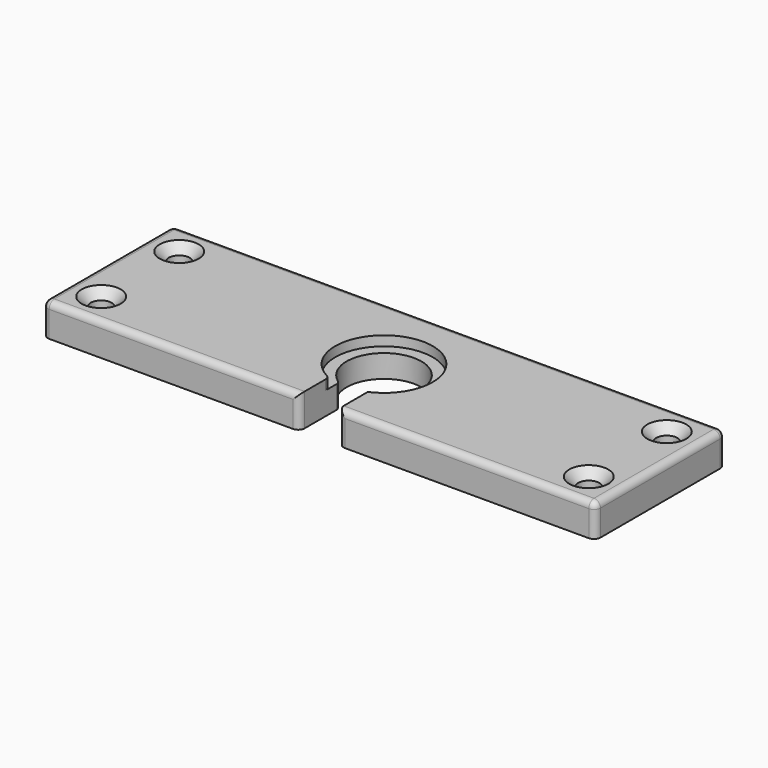
from build123d import *

# Parameters (mm, degrees)
F0_W            = 170
F0_H            = 50
F0_R            = 11.5
F1_DEPTH        = 10
F2_R            = 3.25
F3_DEPTH        = 10.001
F4_R            = 15
F4_R_2          = 11.5
F5_DEPTH        = 3
F7_DEPTH        = 25
F8_T1_DEPTH     = 20.004828627
F8_T3_DEPTH     = 12.3229236974
F8_T5_DEPTH     = 6.1336823274
F9_T1_DEPTH     = 46
F9_T3_DEPTH     = 166
F9_T5_DEPTH     = 13
F9_T7_DEPTH     = 80.0390459698
F9_T9_DEPTH     = 80.0390459698
F9_S13_W        = 2
F9_S13_H        = 2
F9_T14_DEPTH    = 2
F9_S19_W        = 2
F9_S19_H        = 2
F9_T20_DEPTH    = 2
F9_S25_W        = 2
F9_S25_H        = 2
F9_T26_DEPTH    = 2
F9_S31_W        = 2
F9_S31_H        = 2
F9_T32_DEPTH    = 2
F11_D           = 6.5
F11_DEPTH       = 15
F11_CSINK_D     = 12
F11_CSINK_ANGLE = 90
F11_TIP         = 1.9527970118


# Not quite as in the source:
# - a fillet or chamfer that OpenCascade refuses, or shapes differently, is made with other operations: its cross-section is extruded or revolved along the edge and cut away or added


with BuildPart() as f1:
    # F0 (on Top) → F1 (new body)
    with BuildSketch(Plane.XY):
        Rectangle(F0_W, F0_H)
        Circle(F0_R, mode=Mode.SUBTRACT)
    extrude(amount=F1_DEPTH)

    # F2 (on face) → F3 (cut, through all)
    with BuildSketch(Plane.XY.offset(10)):
        with Locations((-75, 15)):
            Circle(F2_R)
        with Locations((-75, -15)):
            Circle(F2_R)
        with Locations((75, -15)):
            Circle(F2_R)
        with Locations((75, 15)):
            Circle(F2_R)
    extrude(amount=-F3_DEPTH, mode=Mode.SUBTRACT)

    # F4 (on face) → F5 (cut)
    with BuildSketch(Plane.XY.offset(10)):
        Circle(F4_R)
        Circle(F4_R_2, mode=Mode.SUBTRACT)
    extrude(amount=-F5_DEPTH, mode=Mode.SUBTRACT)

    # F6 (on face) → F7 (cut)
    with BuildSketch(Plane.XY.offset(10)):
        with BuildLine():
            Line((-6, -13.7477270849), (-6, -25))
            Line((-6, -25), (6, -25))
            Line((6, -25), (6, -13.7477270849))
            ThreePointArc((6, -13.7477270849), (0, -15), (-6, -13.7477270849))
        make_face()
        with BuildLine():
            Line((-6, -9), (-6, -13.7477270849))
            ThreePointArc((-6, -13.7477270849), (0, -15), (6, -13.7477270849))
            Line((6, -13.7477270849), (6, -9))
            Line((6, -9), (-6, -9))
        make_face()
    extrude(amount=-F7_DEPTH, mode=Mode.SUBTRACT)

    # F8: fillet of radius 2 on 5 edges, made by hand

    # F8_s2 → F8_t1 (cut)
    with BuildSketch(Plane.XY.offset(-5.0024143135)):
        with BuildLine():
            ThreePointArc((-5.9996, -22.9990343146), (-6.5857864376, -24.4142135624), (-8.0009656854, -25.0004))
            Line((-8.0009656854, -25.0004), (-8.0009656854, -25.2005365685))
            ThreePointArc((-8.0009656854, -25.2005365685), (-7.0004828427, -25.2001365685), (-6, -25.2001365685))
            Line((-6, -25.2001365685), (-5.7998634315, -25))
            ThreePointArc((-5.7998634315, -25), (-5.7998634315, -23.9995171573), (-5.7994634315, -22.9990343146))
            Line((-5.7994634315, -22.9990343146), (-5.9996, -22.9990343146))
        make_face()
        with BuildLine():
            ThreePointArc((5.9996, -22.9990343146), (6.5857864376, -24.4142135624), (8.0009656854, -25.0004))
            Line((8.0009656854, -25.0004), (8.0009656854, -25.2005365685))
            ThreePointArc((8.0009656854, -25.2005365685), (7.0004828427, -25.2001365685), (6, -25.2001365685))
            Line((6, -25.2001365685), (5.7998634315, -25))
            ThreePointArc((5.7998634315, -25), (5.7998634315, -23.9995171573), (5.7994634315, -22.9990343146))
            Line((5.7994634315, -22.9990343146), (5.9996, -22.9990343146))
        make_face()
    extrude(amount=F8_T1_DEPTH, mode=Mode.SUBTRACT)

    # F8_s4 → F8_t3 (cut)
    with BuildSketch(Plane.XY.offset(-2.6614618487)):
        with BuildLine():
            ThreePointArc((-6.8152717523, -9.2624441214), (-6.215115784, -9.9716058978), (-5.9996, -10.8752930995))
            Line((-5.9996, -10.8752930995), (-5.79936, -10.8752930995))
            ThreePointArc((-5.79936, -10.8752930995), (-5.79976, -10.3430007673), (-5.79976, -9.8107084352))
            Line((-5.79976, -9.8107084352), (-5.8955269565, -9.6398826737))
            ThreePointArc((-5.8955269565, -9.6398826737), (-6.3019268651, -9.3792480426), (-6.6965989276, -9.1011592236))
            Line((-6.6965989276, -9.1011592236), (-6.8152717523, -9.2624441214))
        make_face()
        with BuildLine():
            ThreePointArc((5.9996, -10.8752930995), (6.215115784, -9.9716058978), (6.8152717523, -9.2624441214))
            Line((6.8152717523, -9.2624441214), (6.6965989276, -9.1011592236))
            ThreePointArc((6.6965989276, -9.1011592236), (6.3019268651, -9.3792480426), (5.8955269565, -9.6398826737))
            Line((5.8955269565, -9.6398826737), (5.79976, -9.8107084352))
            ThreePointArc((5.79976, -9.8107084352), (5.79976, -10.3430007673), (5.79936, -10.8752930995))
            Line((5.79936, -10.8752930995), (5.9996, -10.8752930995))
        make_face()
    extrude(amount=F8_T3_DEPTH, mode=Mode.SUBTRACT)

    # F8_s6 → F8_t5 (cut)
    with BuildSketch(Plane.XY.offset(7)):
        with BuildLine():
            ThreePointArc((-7.0595694154, -13.2344429361), (-6.2849198093, -13.9710342475), (-5.9996, -15.001199952))
            Line((-5.9996, -15.001199952), (-5.79936, -15.001199952))
            ThreePointArc((-5.79936, -15.001199952), (-5.79976, -14.3744635184), (-5.79976, -13.7477270849))
            Line((-5.79976, -13.7477270849), (-5.919904, -13.5642040934))
            ThreePointArc((-5.919904, -13.5642040934), (-6.4476696186, -13.3214283223), (-6.9653263569, -13.0577672345))
            Line((-6.9653263569, -13.0577672345), (-7.0595694154, -13.2344429361))
        make_face()
    extrude(amount=F8_T5_DEPTH, mode=Mode.SUBTRACT)

    # F9: fillet of radius 2 on 9 edges, made by hand

    # F9_s2 → F9_t1 (cut)
    with BuildSketch(Plane.XZ.offset(-23)):
        with BuildLine():
            ThreePointArc((-83, 10), (-84.4142135624, 9.4142135624), (-85, 8))
            Line((-85, 8), (-85, 10))
            Line((-85, 10), (-83, 10))
        make_face()
        with BuildLine():
            ThreePointArc((85, 8), (84.4142135624, 9.4142135624), (83, 10))
            Line((83, 10), (85, 10))
            Line((85, 10), (85, 8))
        make_face()
    extrude(amount=F9_T1_DEPTH, mode=Mode.SUBTRACT)

    # F9_s4 → F9_t3 (cut)
    with BuildSketch(Plane.YZ.offset(-83)):
        with BuildLine():
            ThreePointArc((23, 10), (24.4142135624, 9.4142135624), (25, 8))
            Line((25, 8), (25, 10))
            Line((25, 10), (23, 10))
        make_face()
    extrude(amount=F9_T3_DEPTH, mode=Mode.SUBTRACT)

    # F9_s6 → F9_t5 (cut)
    with BuildSketch(Plane.XY.offset(-5)):
        with BuildLine():
            ThreePointArc((85, -23), (84.4142135624, -24.4142135624), (83, -25))
            Line((83, -25), (85, -25))
            Line((85, -25), (85, -23))
        make_face()
        with BuildLine():
            ThreePointArc((85, 23), (84.4142135624, 24.4142135624), (83, 25))
            Line((83, 25), (85, 25))
            Line((85, 25), (85, 23))
        make_face()
        with BuildLine():
            ThreePointArc((-85, -23), (-84.4142135624, -24.4142135624), (-83, -25))
            Line((-83, -25), (-85, -25))
            Line((-85, -25), (-85, -23))
        make_face()
        with BuildLine():
            ThreePointArc((-85, 23), (-84.4142135624, 24.4142135624), (-83, 25))
            Line((-83, 25), (-85, 25))
            Line((-85, 25), (-85, 23))
        make_face()
    extrude(amount=F9_T5_DEPTH, mode=Mode.SUBTRACT)

    # F9_s8 → F9_t7 (cut)
    with BuildSketch(Plane.YZ.offset(2.9609540302)):
        with BuildLine():
            ThreePointArc((-23, 10), (-24.4142135624, 9.4142135624), (-25, 8))
            Line((-25, 8), (-25, 10))
            Line((-25, 10), (-23, 10))
        make_face()
    extrude(amount=F9_T7_DEPTH, mode=Mode.SUBTRACT)

    # F9_s10 → F9_t9 (cut)
    with BuildSketch(Plane.YZ.offset(-83)):
        with BuildLine():
            ThreePointArc((-23, 10), (-24.4142135624, 9.4142135624), (-25, 8))
            Line((-25, 8), (-25, 10))
            Line((-25, 10), (-23, 10))
        make_face()
    extrude(amount=F9_T9_DEPTH, mode=Mode.SUBTRACT)


with BuildPart() as f9_tool12:
    # F9_s13 → F9_t14 (new body)
    with BuildSketch(Plane.XY.offset(8)):
        with Locations((-84, 24)):
            Rectangle(F9_S13_W, F9_S13_H)
    extrude(amount=F9_T14_DEPTH)

    # F9_s15 → F9_t16 (revolve, cut)
    with BuildSketch(Plane(origin=(-83, 23, 8), x_dir=(0.7071067812, -0.7071067812, 0), z_dir=(-0.7071067812, -0.7071067812, 0))):
        with BuildLine():
            ThreePointArc((0, -2), (2, 0), (0, 2))
            Line((0, 2), (0, -2))
        make_face()
    revolve(axis=Axis((-83, 23, 8), (0, 0, 1)), mode=Mode.SUBTRACT)


with BuildPart() as f1_1:
    add(f1.part)

    # F9_t11: cut F9_tool12
    add(f9_tool12.part, mode=Mode.SUBTRACT)


with BuildPart() as f9_tool18:
    # F9_s19 → F9_t20 (new body)
    with BuildSketch(Plane.XY.offset(8)):
        with Locations((-84, -24)):
            Rectangle(F9_S19_W, F9_S19_H)
    extrude(amount=F9_T20_DEPTH)

    # F9_s21 → F9_t22 (revolve, cut)
    with BuildSketch(Plane(origin=(-83, -23, 8), x_dir=(0.7071067812, 0.7071067812, 0), z_dir=(0.7071067812, -0.7071067812, 0))):
        with BuildLine():
            ThreePointArc((0, -2), (2, 0), (0, 2))
            Line((0, 2), (0, -2))
        make_face()
    revolve(axis=Axis((-83, -23, 8), (0, 0, 1)), mode=Mode.SUBTRACT)


with BuildPart() as f1_2:
    add(f1_1.part)

    # F9_t17: cut F9_tool18
    add(f9_tool18.part, mode=Mode.SUBTRACT)


with BuildPart() as f9_tool24:
    # F9_s25 → F9_t26 (new body)
    with BuildSketch(Plane.YZ.offset(83)):
        with Locations((24, 9)):
            Rectangle(F9_S25_W, F9_S25_H)
    extrude(amount=F9_T26_DEPTH)

    # F9_s27 → F9_t28 (revolve, cut)
    with BuildSketch(Plane(origin=(83, 23, 8), x_dir=(0, -0.7071067812, -0.7071067812), z_dir=(0, -0.7071067812, 0.7071067812))):
        with BuildLine():
            ThreePointArc((0, -2), (2, 0), (0, 2))
            Line((0, 2), (0, -2))
        make_face()
    revolve(axis=Axis((83, 23, 8), (1, 0, 0)), mode=Mode.SUBTRACT)


with BuildPart() as f1_3:
    add(f1_2.part)

    # F9_t23: cut F9_tool24
    add(f9_tool24.part, mode=Mode.SUBTRACT)


with BuildPart() as f9_tool30:
    # F9_s31 → F9_t32 (new body)
    with BuildSketch(Plane.YZ.offset(83)):
        with Locations((-24, 9)):
            Rectangle(F9_S31_W, F9_S31_H)
    extrude(amount=F9_T32_DEPTH)

    # F9_s33 → F9_t34 (revolve, cut)
    with BuildSketch(Plane(origin=(83, -23, 8), x_dir=(0, 0.7071067812, -0.7071067812), z_dir=(0, -0.7071067812, -0.7071067812))):
        with BuildLine():
            ThreePointArc((0, -2), (2, 0), (0, 2))
            Line((0, 2), (0, -2))
        make_face()
    revolve(axis=Axis((83, -23, 8), (1, 0, 0)), mode=Mode.SUBTRACT)


with BuildPart() as f1_4:
    add(f1_3.part)

    # F9_t29: cut F9_tool30
    add(f9_tool30.part, mode=Mode.SUBTRACT)

    # F11
    with Locations(Plane.XY.offset(10)):
        with Locations((-75, 15), (-75, -15), (75, -15), (75, 15)):
            CounterSinkHole(F11_D / 2, F11_CSINK_D / 2, depth=F11_DEPTH, counter_sink_angle=F11_CSINK_ANGLE)
            with Locations((0, 0, -(F11_DEPTH + F11_TIP / 2))):  # 118° drill point
                Cone(0, F11_D / 2, F11_TIP, mode=Mode.SUBTRACT)


solid = f1_4.part
